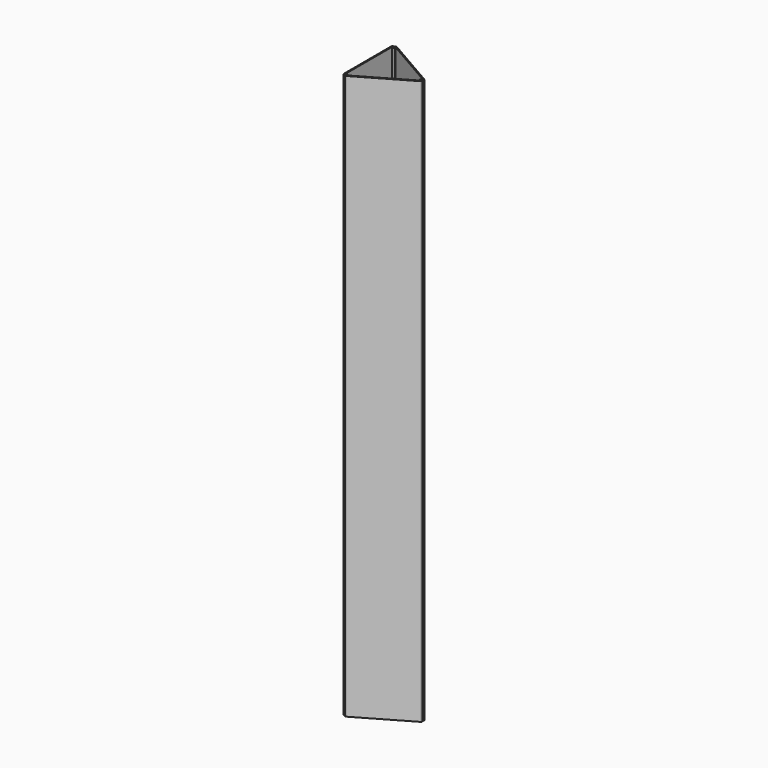
from build123d import *

# Parameters (mm, degrees)
F1_DEPTH    = 2500
F2_T        = 5
F2_T3_DEPTH = 2510
F4_DEPTH    = 2


# Not quite as in the source:
# - a shell that OpenCascade refuses in one call is made with other operations: the cavity is built on its own and cut out


with BuildPart() as f1:
    # F0 (on Top) → F1 (new body)
    with BuildSketch(Plane.XY):
        with BuildLine():
            Line((243.3531384634, 9.5), (16.4544826719, 140.5))
            ThreePointArc((16.4544826719, 140.5), (10.418948766, 139.705406887), (9.624355653, 133.6698729811))
            Line((9.624355653, 133.6698729811), (10.874355653, 131.5048094716))
            Line((10.874355653, 131.5048094716), (10.5801270189, 131.3349364905))
            Line((10.5801270189, 131.3349364905), (9.3301270189, 133.5))
            ThreePointArc((9.3301270189, 133.5), (3.7059047745, 135.8296291314), (0, 131))
            Line((0, 131), (0, -131))
            ThreePointArc((0, -131), (3.7059047745, -135.8296291314), (9.3301270189, -133.5))
            Line((9.3301270189, -133.5), (10.5801270189, -131.3349364905))
            Line((10.5801270189, -131.3349364905), (10.874355653, -131.5048094716))
            Line((10.874355653, -131.5048094716), (9.624355653, -133.6698729811))
            ThreePointArc((9.624355653, -133.6698729811), (10.418948766, -139.705406887), (16.4544826719, -140.5))
            Line((16.4544826719, -140.5), (243.3531384634, -9.5))
            ThreePointArc((243.3531384634, -9.5), (245.6827675949, -3.8757777556), (240.8531384634, -0.1698729811))
            Line((240.8531384634, -0.1698729811), (238.3531384634, -0.1698729811))
            Line((238.3531384634, -0.1698729811), (238.3531384634, 0.1698729811))
            Line((238.3531384634, 0.1698729811), (240.8531384634, 0.1698729811))
            ThreePointArc((240.8531384634, 0.1698729811), (245.6827675949, 3.8757777556), (243.3531384634, 9.5))
        make_face()
    extrude(amount=F1_DEPTH)

    # F2: shell of thickness 5, made by hand


with BuildPart() as f2_core1:
    # F2_t2: copy of F1
    add(f1.part)

    # the walls: a layer under each face that stays
    f2_faces = [f2_core1.faces().sort_by_distance(p)[0] for p in [
        (129.9038105677, 75, 1250),
        (10.249355653, 132.5873412263, 1250),
        (10.727241336, 131.4198729811, 1250),
        (9.9551270189, 132.4174682453, 1250),
        (0, 0, 1250),
        (9.9551270189, -132.4174682453, 1250),
        (10.727241336, -131.4198729811, 1250),
        (10.249355653, -132.5873412263, 1250),
        (129.9038105677, -75, 1250),
        (239.6031384634, -0.1698729811, 1250),
        (238.3531384634, 0, 1250),
        (239.6031384634, 0.1698729811, 1250),
    ]]
    thicken(f2_faces, amount=-F2_T, mode=Mode.SUBTRACT)

    # F2_s4 → F2_t3 (cut)
    with BuildSketch(Plane.XY.offset(-5)):
        Polygon((10.8060543828, 131.5231107418), (15.2044826719, 134.0048094716), (17.7044826719, 129.6746824527), (13.374355653, 127.1746824527), align=None)
        Polygon((10.5984282891, 131.4032377607), (13.0801270189, 127.0048094716), (8.75, 124.5048094716), (6.25, 128.8349364905), align=None)
        Polygon((10.5984282891, -131.4032377607), (6.25, -128.8349364905), (8.75, -124.5048094716), (13.0801270189, -127.0048094716), align=None)
        Polygon((10.8060543828, -131.5231107418), (13.374355653, -127.1746824527), (17.7044826719, -129.6746824527), (15.2044826719, -134.0048094716), align=None)
        Polygon((238.4031384634, -0.1198729811), (238.3531384634, -5.1698729811), (233.3531384634, -5.1698729811), (233.3531384634, -0.1698729811), align=None)
        Polygon((238.4031384634, 0.1198729811), (233.3531384634, 0.1698729811), (233.3531384634, 5.1698729811), (238.3531384634, 5.1698729811), align=None)
    extrude(amount=F2_T3_DEPTH, mode=Mode.SUBTRACT)


with BuildPart() as f1_1:
    add(f1.part)

    # what is left inside the walls is the cavity
    f2_cavity = [f2_core1.part.solids().sort_by_distance(p)[0] for p in [
        (5.05, 0, 1666.666667),
    ]]
    add(f2_cavity, mode=Mode.SUBTRACT)

    # F3 (on face) → F4 (join)
    with BuildSketch(Plane(origin=(0, 0, 0), x_dir=(1, 0, 0), z_dir=(0, 0, -1))):
        Polygon((8.75, 124.5048094716), (5, 131), (5, -131), (8.75, -124.5048094716), (17.7044826719, -129.6746824527), (13.9544826719, -136.1698729811), (240.8531384634, -5.1698729811), (233.3531384634, -5.1698729811), (233.3531384634, 5.1698729811), (240.8531384634, 5.1698729811), (13.9544826719, 136.1698729811), (17.7044826719, 129.6746824527), align=None)
    extrude(amount=-F4_DEPTH)


solid = f1_1.part
